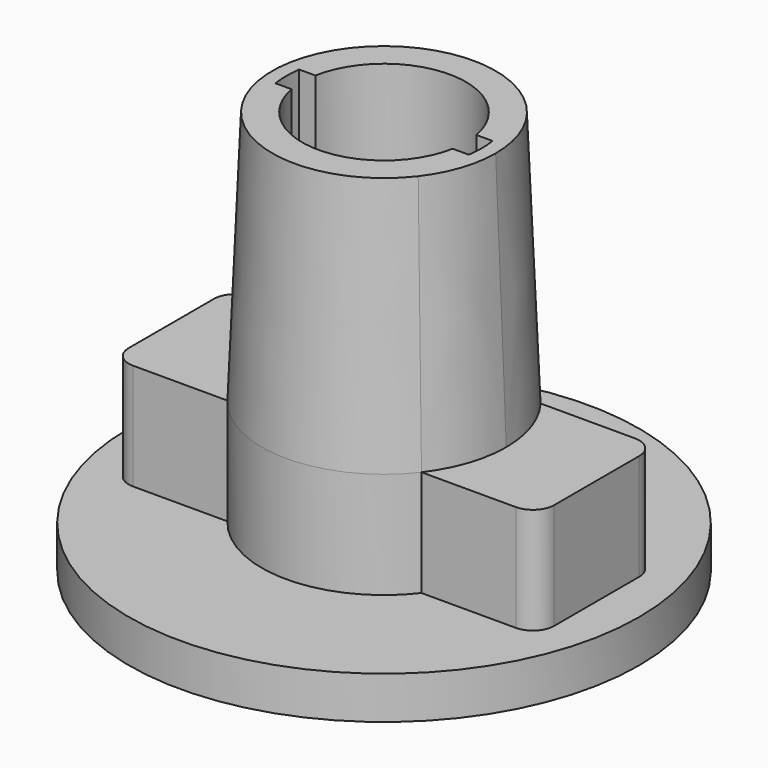
from build123d import *

# Parameters (mm, degrees)
F0_R     = 12
F0_R_2   = 3.75
F1_DEPTH = 2
F3_DEPTH = 5
F5_DEPTH = 12
F6_SIZE2 = 11.99999
F6_SIZE  = 0.49999


# Not quite as in the source:
# - a fillet or chamfer is up to 0.001 mm smaller than in the source, because OpenCascade refuses the exact size


with BuildPart() as f1:
    # F0 (on Top) → F1 (new body)
    with BuildSketch(Plane.XY):
        Circle(F0_R)
        Circle(F0_R_2, mode=Mode.SUBTRACT)
    extrude(amount=F1_DEPTH)

    # F2 (on face) → F3 (join)
    with BuildSketch(Plane.XY.offset(2)):
        with BuildLine():
            Line((-9, -3.5), (-4.5620718977, -3.5))
            ThreePointArc((-4.5620718977, -3.5), (-5.75, 0), (-4.5620718977, 3.5))
            Line((-4.5620718977, 3.5), (-9, 3.5))
            ThreePointArc((-9, 3.5), (-9.7071067812, 3.2071067812), (-10, 2.5))
            Line((-10, 2.5), (-10, 0))
            Line((-10, 0), (-10, -2.5))
            ThreePointArc((-10, -2.5), (-9.7071067812, -3.2071067812), (-9, -3.5))
        make_face()
        with BuildLine():
            Line((-4.5620718977, -3.5), (-1.6039014932, -3.5))
            ThreePointArc((-1.6039014932, -3.5), (-3.0368237131, -2.3664745373), (-3.7858288392, -0.7))
            Line((-3.7858288392, -0.7), (-4, -0.7))
            Line((-4, -0.7), (-4.5464271687, -0.7))
            ThreePointArc((-4.5464271687, -0.7), (-4.6, 0), (-4.5464271687, 0.7))
            Line((-4.5464271687, 0.7), (-3.7858288392, 0.7))
            ThreePointArc((-3.7858288392, 0.7), (-3.0368237131, 2.3664745373), (-1.6039014932, 3.5))
            Line((-1.6039014932, 3.5), (-4.5620718977, 3.5))
            ThreePointArc((-4.5620718977, 3.5), (-5.75, 0), (-4.5620718977, -3.5))
        make_face()
        with BuildLine():
            Line((4.5620718977, -3.5), (1.6039014932, -3.5))
            ThreePointArc((1.6039014932, -3.5), (0, -3.85), (-1.6039014932, -3.5))
            Line((-1.6039014932, -3.5), (-4.5620718977, -3.5))
            ThreePointArc((-4.5620718977, -3.5), (0, -5.75), (4.5620718977, -3.5))
        make_face()
        with BuildLine():
            ThreePointArc((5.75, 0), (5.4449248577, -1.8480512152), (4.5620718977, -3.5))
            Line((4.5620718977, -3.5), (9, -3.5))
            ThreePointArc((9, -3.5), (9.7071067812, -3.2071067812), (10, -2.5))
            Line((10, -2.5), (10, 0))
            Line((10, 0), (10, 2.5))
            ThreePointArc((10, 2.5), (9.7071067812, 3.2071067812), (9, 3.5))
            Line((9, 3.5), (4.5620718977, 3.5))
            ThreePointArc((4.5620718977, 3.5), (5.4449248577, 1.8480512152), (5.75, 0))
        make_face()
        with BuildLine():
            ThreePointArc((3.7858288392, -0.7), (3.0368237131, -2.3664745373), (1.6039014932, -3.5))
            Line((1.6039014932, -3.5), (4.5620718977, -3.5))
            ThreePointArc((4.5620718977, -3.5), (5.4449248577, -1.8480512152), (5.75, 0))
            ThreePointArc((5.75, 0), (5.4449248577, 1.8480512152), (4.5620718977, 3.5))
            Line((4.5620718977, 3.5), (1.6039014932, 3.5))
            ThreePointArc((1.6039014932, 3.5), (3.0368237131, 2.3664745373), (3.7858288392, 0.7))
            Line((3.7858288392, 0.7), (4.5464271687, 0.7))
            ThreePointArc((4.5464271687, 0.7), (4.6, 0), (4.5464271687, -0.7))
            Line((4.5464271687, -0.7), (4, -0.7))
            Line((4, -0.7), (3.7858288392, -0.7))
        make_face()
        with BuildLine():
            Line((-4.5620718977, 3.5), (-1.6039014932, 3.5))
            ThreePointArc((-1.6039014932, 3.5), (0, 3.85), (1.6039014932, 3.5))
            Line((1.6039014932, 3.5), (4.5620718977, 3.5))
            ThreePointArc((4.5620718977, 3.5), (0, 5.75), (-4.5620718977, 3.5))
        make_face()
    extrude(amount=F3_DEPTH)

    # F4 (on face) → F5 (join)
    with BuildSketch(Plane.XY.offset(7)):
        with BuildLine():
            ThreePointArc((4.5620718977, -3.5), (5.4449248577, -1.8480512152), (5.75, 0))
            ThreePointArc((5.75, 0), (5.4449248577, 1.8480512152), (4.5620718977, 3.5))
            ThreePointArc((4.5620718977, 3.5), (0, 5.75), (-4.5620718977, 3.5))
            ThreePointArc((-4.5620718977, 3.5), (-5.75, 0), (-4.5620718977, -3.5))
            ThreePointArc((-4.5620718977, -3.5), (0, -5.75), (4.5620718977, -3.5))
        make_face()
        with BuildLine():
            ThreePointArc((-3.7858288392, 0.7), (0, 3.85), (3.7858288392, 0.7))
            Line((3.7858288392, 0.7), (4.5464271687, 0.7))
            ThreePointArc((4.5464271687, 0.7), (4.6, 0), (4.5464271687, -0.7))
            Line((4.5464271687, -0.7), (3.7858288392, -0.7))
            ThreePointArc((3.7858288392, -0.7), (0, -3.85), (-3.7858288392, -0.7))
            Line((-3.7858288392, -0.7), (-4.5464271687, -0.7))
            ThreePointArc((-4.5464271687, -0.7), (-4.6, 0), (-4.5464271687, 0.7))
            Line((-4.5464271687, 0.7), (-3.7858288392, 0.7))
        make_face(mode=Mode.SUBTRACT)
    extrude(amount=F5_DEPTH)

    # F6 (size 0.5 and 12 in the source; OpenCascade refuses exactly that, so slightly less here)
    f6_edges = [f1.edges().sort_by_distance(p)[0] for p in [
        (-4.562072, -3.5, 19),
    ]]
    f6_side = f1.faces().sort_by_distance((-4.433037, -3.401005, 19))[0]
    chamfer(f6_edges, length=F6_SIZE, length2=F6_SIZE2, reference=f6_side)


solid = f1.part
